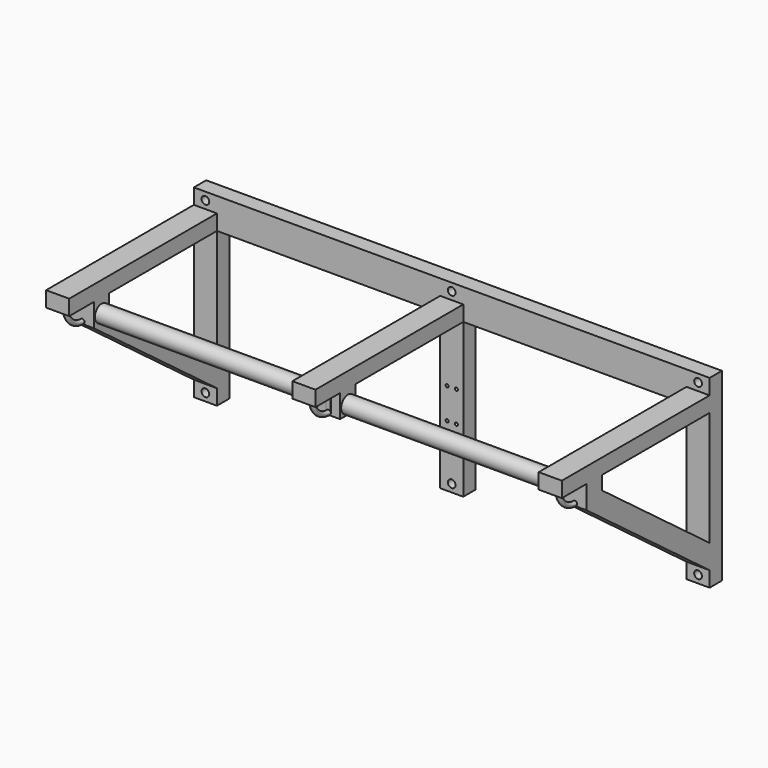
from build123d import *

# Parameters (mm, degrees)
F0_W           = 38.1
F0_H           = 254
F0_H_2         = 25.4
F0_W_2         = 368.3
F1_DEPTH       = 25.4
F2_W           = 38.1
F2_H           = 25.4
F3_DEPTH       = 304.8
F4_W           = 850.9
F4_H           = 25.4
F5_DEPTH       = 25.4
F7_DEPTH       = 38.1
F9_DEPTH       = 38.1
F10_W          = 31.75
F10_H          = 38.1
F11_DEPTH      = 38.1
F12_R          = 2.54
F13_DEPTH      = 12.7
F14_R          = 13.97
F15_DEPTH      = 406.4
F15_DEPTH_BACK = 406.4
F17_DEPTH      = 38.1
F19_DEPTH      = 38.1
F21_DEPTH      = 38.1
F22_W          = 15.24
F22_H          = 39.0179467559
F23_DEPTH      = 50.8
F24_W          = 15.24
F24_H          = 39.0179467559
F25_DEPTH      = 50.8
F26_W          = 15.24
F26_H          = 39.0179467559
F27_DEPTH      = 50.8
F28_R          = 3.80999
F29_R          = 3.81
F30_DEPTH      = 25.4
F31_R          = 6.35
F32_DEPTH      = 12.7
F33_R          = 6.35
F34_DEPTH      = 12.7
F35_R          = 6.35
F36_DEPTH      = 12.7
F37_R          = 6.35
F38_DEPTH      = 12.7


# Not quite as in the source:
# - a fillet or chamfer is up to 0.001 mm smaller than in the source, because OpenCascade refuses the exact size


with BuildPart() as f1:
    # F0 (on Front) → F1 (new body)
    with BuildSketch(Plane.XZ):
        with Locations((0, -25.4)):
            Rectangle(F0_W, F0_H)
        with Locations((0, 114.3)):
            Rectangle(F0_W, F0_H_2)
        with Locations((203.2, 114.3)):
            Rectangle(F0_W_2, F0_H_2)
        with Locations((-203.2, 114.3)):
            Rectangle(F0_W_2, F0_H_2)
        with Locations((0, 139.7)):
            Rectangle(F0_W, F0_H_2)
        with Locations((406.4, -25.4)):
            Rectangle(F0_W, F0_H)
        with Locations((406.4, 114.3)):
            Rectangle(F0_W, F0_H_2)
        with Locations((-406.4, 114.3)):
            Rectangle(F0_W, F0_H_2)
        with Locations((-406.4, -25.4)):
            Rectangle(F0_W, F0_H)
        with Locations((406.4, 139.7)):
            Rectangle(F0_W, F0_H_2)
        with Locations((-406.4, 139.7)):
            Rectangle(F0_W, F0_H_2)
    extrude(amount=F1_DEPTH)

    # F2 (on face) → F3 (join)
    with BuildSketch(Plane.XZ.offset(25.4)):
        with Locations((-406.4, 114.3)):
            Rectangle(F2_W, F2_H)
        with Locations((0, 114.3)):
            Rectangle(F2_W, F2_H)
        with Locations((406.4, 114.3)):
            Rectangle(F2_W, F2_H)
    extrude(amount=F3_DEPTH)

    # F4 (on face) → F5 (join)
    with BuildSketch(Plane.XZ.offset(25.4)):
        with Locations((0, 139.7)):
            Rectangle(F4_W, F4_H)
    extrude(amount=-F5_DEPTH)

    # F6 (on face) → F7 (join)
    with BuildSketch(Plane.YZ.offset(425.45)):
        Polygon((-279.4, 63.5), (-25.4, -127), (-25.4, -87.3125), (-247.65, 79.375), (-247.65, 101.6), (-279.4, 101.6), align=None)
    extrude(amount=-F7_DEPTH)

    # F8 (on face) → F9 (join)
    with BuildSketch(Plane.YZ.offset(-387.35)):
        Polygon((-279.4, 63.5), (-25.4, -127), (-25.4, -87.3125), (-247.65, 79.375), (-247.65, 101.6), (-279.4, 101.6), align=None)
    extrude(amount=-F9_DEPTH)

    # F10 (on face) → F11 (join)
    with BuildSketch(Plane.YZ.offset(19.05)):
        with Locations((-263.8239381313, 82.55)):
            Rectangle(F10_W, F10_H)
    extrude(amount=-F11_DEPTH)

    # F12 (on face) → F13 (cut)
    with BuildSketch(Plane.XZ.offset(25.4)):
        with Locations((-7.62, 0)):
            Circle(F12_R)
        with Locations((7.62, 0)):
            Circle(F12_R)
        with Locations((-7.62, -50.8)):
            Circle(F12_R)
        with Locations((7.62, -50.8)):
            Circle(F12_R)
    extrude(amount=-F13_DEPTH, mode=Mode.SUBTRACT)

    # F14 (on Right) → F15 (join, two sides)
    with BuildSketch(Plane.YZ) as f15_sk:
        with Locations((-263.2673084736, 78.74)):
            Circle(F14_R)
    extrude(amount=-F15_DEPTH)
    extrude(f15_sk.sketch, amount=F15_DEPTH_BACK)

    # F16 (on face) → F17 (join)
    with BuildSketch(Plane(origin=(-425.45, 0, 0), x_dir=(0, -1, 0), z_dir=(-1, 0, 0))):
        with BuildLine():
            Line((279.4, 71.12), (279.4, 63.5))
            ThreePointArc((279.4, 63.5), (306.3407683632, 74.6592316368), (317.5, 101.6))
            Line((317.5, 101.6), (309.88, 101.6))
            ThreePointArc((309.88, 101.6), (300.9526146906, 80.0473853094), (279.4, 71.12))
        make_face()
    extrude(amount=-F17_DEPTH)

    # F18 (on face) → F19 (join)
    with BuildSketch(Plane(origin=(-19.05, 0, 0), x_dir=(0, -1, 0), z_dir=(-1, 0, 0))):
        with BuildLine():
            Line((279.6989381313, 71.12), (279.6989381313, 63.5))
            ThreePointArc((279.6989381313, 63.5), (306.6397064945, 74.6592316368), (317.7989381313, 101.6))
            Line((317.7989381313, 101.6), (310.1789381313, 101.6))
            ThreePointArc((310.1789381313, 101.6), (301.2515528219, 80.0473853094), (279.6989381313, 71.12))
        make_face()
    extrude(amount=-F19_DEPTH)

    # F20 (on face) → F21 (join)
    with BuildSketch(Plane(origin=(387.35, 0, 0), x_dir=(0, -1, 0), z_dir=(-1, 0, 0))):
        with BuildLine():
            Line((279.4, 71.12), (279.4, 63.5))
            ThreePointArc((279.4, 63.5), (306.3407683632, 74.6592316368), (317.5, 101.6))
            Line((317.5, 101.6), (309.88, 101.6))
            ThreePointArc((309.88, 101.6), (300.9526146906, 80.0473853094), (279.4, 71.12))
        make_face()
    extrude(amount=-F21_DEPTH)

    # F22 (on face) → F23 (cut)
    with BuildSketch(Plane.XZ.offset(330.2)):
        with Locations((-417.83, 82.0910266221)):
            Rectangle(F22_W, F22_H)
        with Locations((-394.97, 82.0910266221)):
            Rectangle(F22_W, F22_H)
    extrude(amount=-F23_DEPTH, mode=Mode.SUBTRACT)

    # F24 (on face) → F25 (cut)
    with BuildSketch(Plane.XZ.offset(330.2)):
        with Locations((-11.43, 82.0910266221)):
            Rectangle(F24_W, F24_H)
        with Locations((11.43, 82.0910266221)):
            Rectangle(F24_W, F24_H)
    extrude(amount=-F25_DEPTH, mode=Mode.SUBTRACT)

    # F26 (on face) → F27 (cut)
    with BuildSketch(Plane.XZ.offset(330.2)):
        with Locations((394.97, 82.0910266221)):
            Rectangle(F26_W, F26_H)
        with Locations((417.83, 82.0910266221)):
            Rectangle(F26_W, F26_H)
    extrude(amount=-F27_DEPTH, mode=Mode.SUBTRACT)

    # F28 (radius 3.81 in the source; OpenCascade refuses exactly that, so slightly less here)
    f28_edges = [f1.edges().sort_by_distance(p)[0] for p in [
        (402.59, -306.340768, 74.659232),
        (402.59, -300.952615, 80.047385),
        (410.21, -306.340768, 74.659232),
        (410.21, -300.952615, 80.047385),
        (3.81, -301.251553, 80.047385),
        (3.81, -306.639706, 74.659232),
        (-3.81, -301.251553, 80.047385),
        (-3.81, -306.639706, 74.659232),
        (-410.21, -300.952615, 80.047385),
        (-410.21, -306.340768, 74.659232),
        (-402.59, -300.952615, 80.047385),
        (-402.59, -306.340768, 74.659232),
    ]]
    fillet(f28_edges, radius=F28_R)

    # F29 (on face) → F30 (cut)
    with BuildSketch(Plane(origin=(0, 0, 0), x_dir=(-1, 0, 0), z_dir=(0, 1, 0))):
        with Locations((0, -139.7)):
            Circle(F29_R)
        with Locations((0, 139.7)):
            Circle(F29_R)
        with Locations((-406.4, 139.7)):
            Circle(F29_R)
        with Locations((-406.4, -139.7)):
            Circle(F29_R)
        with Locations((406.4, -139.7)):
            Circle(F29_R)
        with Locations((406.4, 139.7)):
            Circle(F29_R)
    extrude(amount=-F30_DEPTH, mode=Mode.SUBTRACT)

    # F31 (on face) → F32 (cut)
    with BuildSketch(Plane.XZ.offset(25.4)):
        with Locations((-406.4, 139.7)):
            Circle(F31_R)
        with Locations((0, 139.7)):
            Circle(F31_R)
        with Locations((406.4, 139.7)):
            Circle(F31_R)
    extrude(amount=-F32_DEPTH, mode=Mode.SUBTRACT)

    # F33 (on face) → F34 (cut)
    with BuildSketch(Plane.XZ.offset(25.4)):
        with Locations((-406.4, -139.7)):
            Circle(F33_R)
    extrude(amount=-F34_DEPTH, mode=Mode.SUBTRACT)

    # F35 (on face) → F36 (cut)
    with BuildSketch(Plane.XZ.offset(25.4)):
        with Locations((0, -139.7)):
            Circle(F35_R)
    extrude(amount=-F36_DEPTH, mode=Mode.SUBTRACT)

    # F37 (on face) → F38 (cut)
    with BuildSketch(Plane.XZ.offset(25.4)):
        with Locations((406.4, -139.7)):
            Circle(F37_R)
    extrude(amount=-F38_DEPTH, mode=Mode.SUBTRACT)


solid = f1.part
